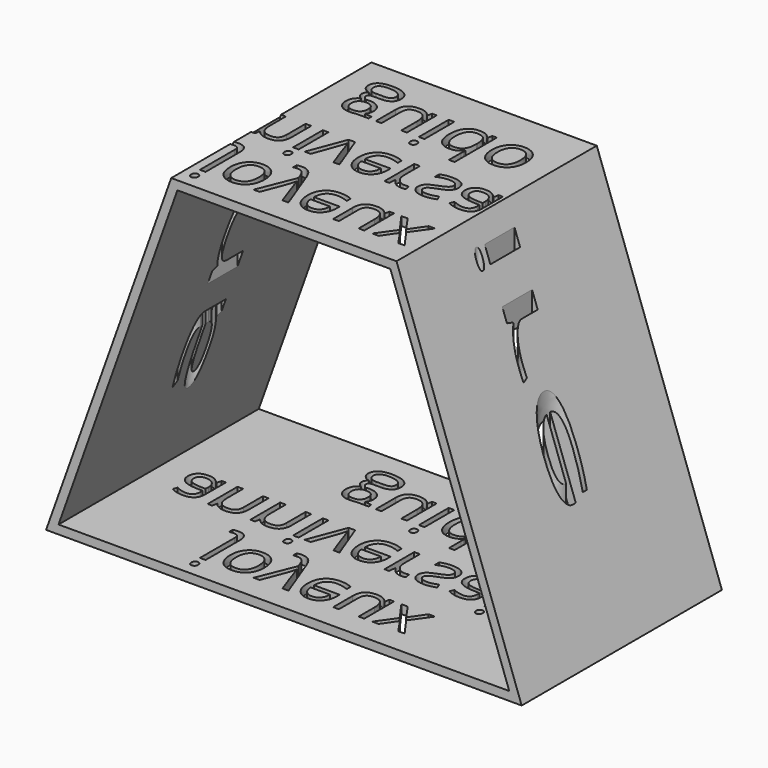
from build123d import *

# Parameters (mm, degrees)
F1_DEPTH     = 100
F2_T         = -3.5
F3_TEXT_SIZE = 27.7777777778
F4_TEXT_SIZE = 27.7777777778
F5_TEXT_SIZE = 27.7777777778
F6_DEPTH     = 140.001


# Not quite as in the source:
# - Text() gives the source's letters only with a copy of the font that has no kerning and outlines rounded to 1/6400 em; it was checked with that copy


with BuildPart() as f1:
    # F0 (on Front) → F1 (new body)
    with BuildSketch(Plane.XZ):
        Polygon((-95, 0), (95, 0), (45, 140), (-45, 140), align=None)
    extrude(amount=F1_DEPTH)

    # F2
    f2_openings = [f1.faces().sort_by_distance(p)[0] for p in [
        (0, -100, 61.666667),
        (0, 0, 61.666667),
    ]]
    offset(amount=F2_T, openings=f2_openings)

    # F3 (on face) + F4 (on face) + F5 (on face) → F6 (cut, through all)
    with BuildSketch(Plane(origin=(0, 0, 0), x_dir=(1, 0, 0), z_dir=(0, 0, -1))):
        with Locations((-43.8715277778, 75.2118310797)):
            Text('joyeux', F3_TEXT_SIZE, font='Open Sans', text_align=(TextAlign.LEFT, TextAlign.BOTTOM))
    with BuildSketch(Plane(origin=(0, 0, 0), x_dir=(1, 0, 0), z_dir=(0, 0, -1))):
        with Locations((-80.2061631944, 45.2118310797)):
            Text('anniversaire', F4_TEXT_SIZE, font='Open Sans', text_align=(TextAlign.LEFT, TextAlign.BOTTOM))
    with BuildSketch(Plane(origin=(0, 0, 0), x_dir=(1, 0, 0), z_dir=(0, 0, -1))):
        with Locations((-36.6666666667, 15.2118310797)):
            Text('guido', F5_TEXT_SIZE, font='Open Sans', text_align=(TextAlign.LEFT, TextAlign.BOTTOM))
    extrude(amount=-F6_DEPTH, mode=Mode.SUBTRACT)


solid = f1.part
